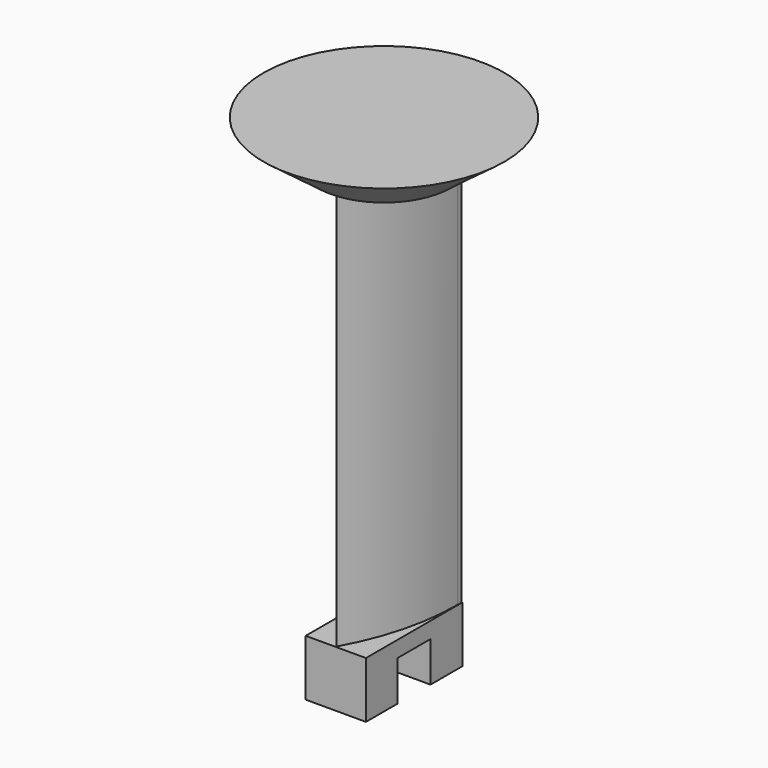
from build123d import *

# Parameters (mm, degrees)
F0_W            = 7.5
F0_H            = 15
F1_DEPTH        = 7
F2_W            = 7.5
F2_H            = 5.1
F3_DEPTH        = 5
F4_W            = 7.4
F4_H            = 14.9
F5_DEPTH        = 50
F6_R            = 15
F6_W            = 7.4
F6_H            = 14.9
F7_DEPTH        = 5
F8_SIZE2        = 6.635214
F8_SIZE         = 4.99999
F9_T1_DEPTH     = 50
F10_T1_DEPTH    = 50
F12_D           = 2.5
F12_DEPTH       = 15
F12_CSINK_D     = 4
F12_CSINK_ANGLE = 90
F12_TIP         = 0.7510757738


# Not quite as in the source:
# - a fillet or chamfer that OpenCascade refuses, or shapes differently, is made with other operations: its cross-section is extruded or revolved along the edge and cut away or added
# - a fillet or chamfer is up to 0.001 mm smaller than in the source, because OpenCascade refuses the exact size


with BuildPart() as f1:
    # F0 (on Top) → F1 (new body)
    with BuildSketch(Plane.XY):
        Rectangle(F0_W, F0_H)
    extrude(amount=F1_DEPTH)

    # F2 (on face) → F3 (cut)
    with BuildSketch(Plane(origin=(0, 0, 0), x_dir=(1, 0, 0), z_dir=(0, 0, -1))):
        Rectangle(F2_W, F2_H)
    extrude(amount=-F3_DEPTH, mode=Mode.SUBTRACT)

    # F4 (on face) → F5 (join)
    with BuildSketch(Plane.XY.offset(7)):
        Rectangle(F4_W, F4_H)
    extrude(amount=F5_DEPTH)

    # F6 (on face) → F7 (join)
    with BuildSketch(Plane.XY.offset(57)):
        Circle(F6_R)
        Rectangle(F6_W, F6_H, mode=Mode.SUBTRACT)
        Rectangle(F6_W, F6_H)
    extrude(amount=F7_DEPTH)

    # F8 (size 5 and 6.6352241081 in the source; OpenCascade refuses exactly that, so slightly less here)
    f8_edges = [f1.edges().sort_by_distance(p)[0] for p in [
        (-15, 0, 57),
    ]]
    f8_side = f1.faces().sort_by_distance((-15, 0, 59.5))[0]
    chamfer(f8_edges, length=F8_SIZE, length2=F8_SIZE2, reference=f8_side)

    # F9: chamfer of 3.75 on 2 edges, made by hand

    # F9_s2 → F9_t1 (cut)
    with BuildSketch(Plane.XY.offset(7)):
        Polygon((-3.7, -3.7), (0.05, -7.45), (-3.7, -7.45), align=None)
        Polygon((-0.05, -7.45), (3.7, -3.7), (3.7, -7.45), align=None)
    extrude(amount=F9_T1_DEPTH, mode=Mode.SUBTRACT)

    # F10: fillet of radius 29.1289708429 on 2 edges, made by hand

    # F10_s2 → F10_t1 (cut)
    with BuildSketch(Plane.XY.offset(7)):
        with BuildLine():
            ThreePointArc((-3.7, 6.8078986566), (-2.7598273987, -0.5329865801), (0, -7.4))
            Line((0, -7.4), (-3.7, -3.7))
            Line((-3.7, -3.7), (-3.7, 6.8078986566))
        make_face()
        with BuildLine():
            ThreePointArc((3.7, 6.8078986566), (2.7598273987, -0.5329865801), (0, -7.4))
            Line((0, -7.4), (3.7, -3.7))
            Line((3.7, -3.7), (3.7, 6.8078986566))
        make_face()
    extrude(amount=F10_T1_DEPTH, mode=Mode.SUBTRACT)

    # F12
    with Locations(Plane(origin=(0, 0, 5), x_dir=(1, 0, 0), z_dir=(0, 0, -1))):
        with Locations((0, 0)):
            CounterSinkHole(F12_D / 2, F12_CSINK_D / 2, depth=F12_DEPTH, counter_sink_angle=F12_CSINK_ANGLE)
            with Locations((0, 0, -(F12_DEPTH + F12_TIP / 2))):  # 118° drill point
                Cone(0, F12_D / 2, F12_TIP, mode=Mode.SUBTRACT)


solid = f1.part
